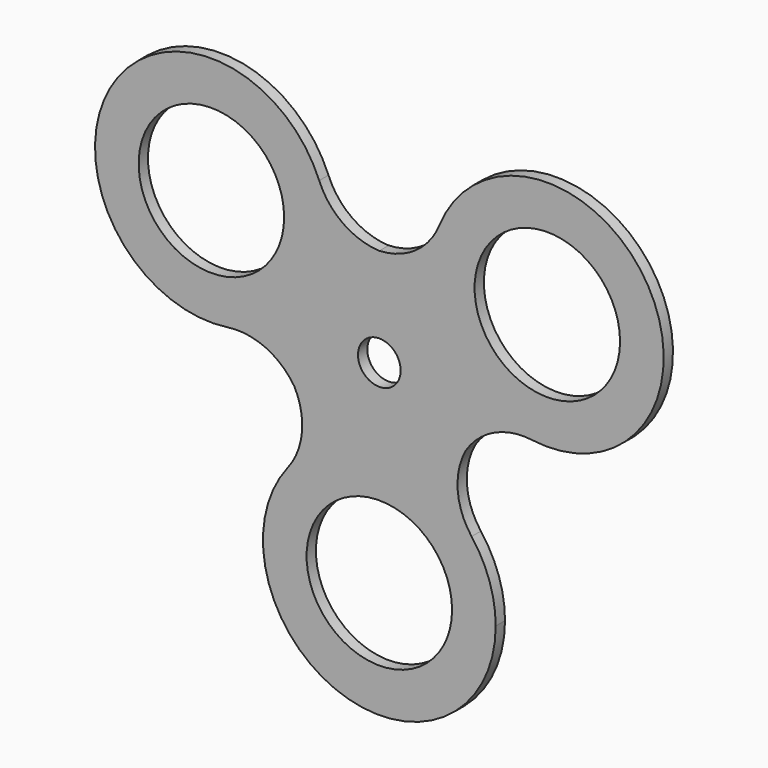
from build123d import *

# Parameters (mm, degrees)
F0_R        = 37.5
F0_R_2      = 11
F1_DEPTH    = 6
F2_T1_DEPTH = 6


# Not quite as in the source:
# - a fillet or chamfer that OpenCascade refuses, or shapes differently, is made with other operations: its cross-section is extruded or revolved along the edge and cut away or added


with BuildPart() as f1:
    # F0 (on Front) → F1 (new body)
    with BuildSketch(Plane.XZ):
        with BuildLine():
            ThreePointArc((57.8643034804, -2.6875543668), (117.2345315762, -1.6261715812), (146.617452556, 49.9741624513))
            ThreePointArc((146.617452556, 49.9741624513), (87.0017930869, 109.9729314583), (26.6223764775, 50.7428277423))
            ThreePointArc((26.6223764775, 50.7428277423), (34.8220541109, 19.6882465841), (57.8643034804, -2.6875543668))
        make_face()
        with Locations((86.617452556, 49.9741624513)):
            Circle(F0_R, mode=Mode.SUBTRACT)
        with BuildLine():
            ThreePointArc((-26.5950813994, 50.0129171058), (-26.5961913872, 50.3778791758), (-26.5995213098, 50.7428277423))
            ThreePointArc((-26.5995213098, 50.7428277423), (-138.5810142586, 79.97060034), (-57.1442597977, -2.261829254))
            ThreePointArc((-57.1442597977, -2.261829254), (-34.7923339042, 19.7395731883), (-26.5950813994, 50.0129171058))
        make_face()
        with Locations((-86.5950813994, 50.0129171058)):
            Circle(F0_R, mode=Mode.SUBTRACT)
        with BuildLine():
            ThreePointArc((57.8643034804, -2.6875543668), (34.8220541109, 19.6882465841), (26.6223764775, 50.7428277423))
            Line((26.6223764775, 50.7428277423), (-26.5995213098, 50.7428277423))
            ThreePointArc((-26.5995213098, 50.7428277423), (-26.5961913872, 50.3778791758), (-26.5950813994, 50.0129171058))
            ThreePointArc((-26.5950813994, 50.0129171058), (-34.7923339042, 19.7395731883), (-57.1442597977, -2.261829254))
            Line((-57.1442597977, -2.261829254), (-30.1904821111, -48.1489171772))
            ThreePointArc((-30.1904821111, -48.1489171772), (0.418102689, -40.0014567665), (30.9101684744, -48.5746999534))
            Line((30.9101684744, -48.5746999534), (57.8643034804, -2.6875543668))
        make_face()
        Circle(F0_R_2, mode=Mode.SUBTRACT)
        with BuildLine():
            ThreePointArc((60, -100), (52.2236062929, -70.4585893064), (30.9101684744, -48.5746999534))
            ThreePointArc((30.9101684744, -48.5746999534), (0.418102689, -40.0014567665), (-30.1904821111, -48.1489171772))
            ThreePointArc((-30.1904821111, -48.1489171772), (-29.9046072816, -152.0164826121), (60, -100))
        make_face()
        with Locations((0, -100)):
            Circle(F0_R, mode=Mode.SUBTRACT)
    extrude(amount=F1_DEPTH)

    # F2: fillet of radius 35 on 6 edges, made by hand

    # F2_s2 → F2_t1 (join)
    with BuildSketch(Plane.XZ):
        with BuildLine():
            ThreePointArc((-44.5789786986, -23.6534191556), (-39.8361716067, -43.7215717477), (-47.2154351555, -62.9769979192))
            ThreePointArc((-47.2154351555, -62.9769979192), (-39.40668727, -54.7549671411), (-30.1904821111, -48.1489171772))
            Line((-30.1904821111, -48.1489171772), (-44.5789786986, -23.6534191556))
        make_face()
        with BuildLine():
            ThreePointArc((-1.3916525599, 50.7428277423), (18.1502571968, 56.7064064225), (31.0327545881, 72.5648984246))
            ThreePointArc((31.0327545881, 72.5648984246), (27.8065544641, 61.8602158597), (26.6223764775, 50.7428277423))
            Line((26.6223764775, 50.7428277423), (-1.3916525599, 50.7428277423))
        make_face()
        with BuildLine():
            ThreePointArc((1.4297644449, 50.7428277423), (-18.1185373349, 56.7107093642), (-31.0004419188, 72.5791764552))
            ThreePointArc((-31.0004419188, 72.5791764552), (-27.7777362498, 61.8670265011), (-26.5995213098, 50.7428277423))
            Line((-26.5995213098, 50.7428277423), (1.4297644449, 50.7428277423))
        make_face()
        with BuildLine():
            ThreePointArc((43.89611258, -26.4672233966), (58.7364313951, -12.7341703185), (78.6957856647, -9.500598529))
            ThreePointArc((78.6957856647, -9.500598529), (67.9663152116, -7.0533315824), (57.8643034804, -2.6875543668))
            Line((57.8643034804, -2.6875543668), (43.89611258, -26.4672233966))
        make_face()
        with BuildLine():
            ThreePointArc((47.5642084271, -63.4261558392), (40.3776870322, -44.2671300594), (45.1312959448, -24.3644277078))
            Line((45.1312959448, -24.3644277078), (30.9101684744, -48.5746999534))
            ThreePointArc((30.9101684744, -48.5746999534), (39.9336749248, -55.2194059106), (47.5642084271, -63.4261558392))
        make_face()
        with BuildLine():
            ThreePointArc((-78.1330690057, -9.3873720033), (-58.0015888855, -12.5081469238), (-43.0181014785, -26.3107131005))
            Line((-43.0181014785, -26.3107131005), (-57.1442597977, -2.261829254))
            ThreePointArc((-57.1442597977, -2.261829254), (-67.3067666659, -6.8022297719), (-78.1330690057, -9.3873720033))
        make_face()
    extrude(amount=F2_T1_DEPTH)


solid = f1.part
